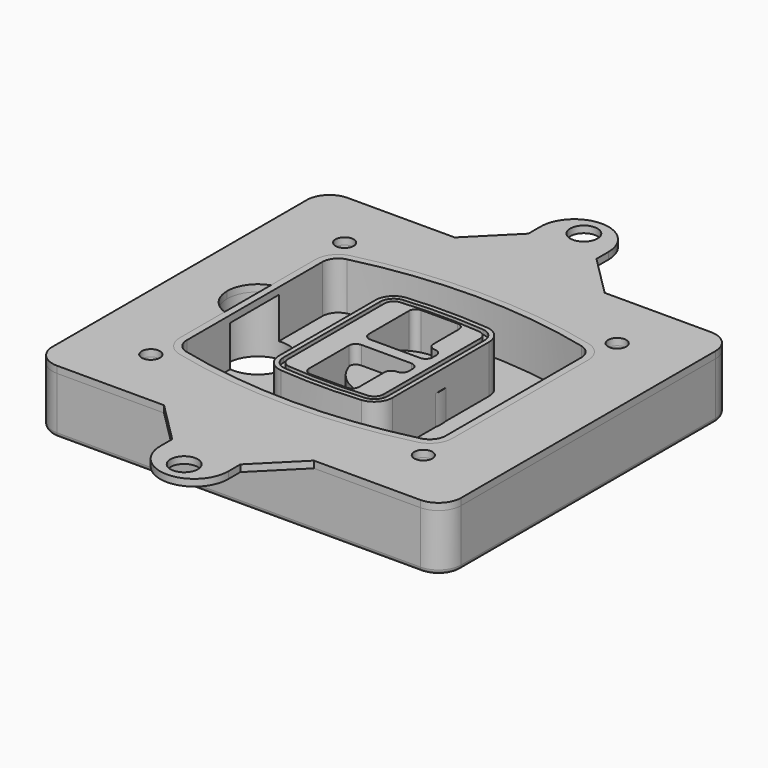
from build123d import *

# Parameters (mm, degrees)
F0_R      = 4
F1_DEPTH  = 25
F2_DEPTH  = 3
F3_DEPTH  = 18
F5_DEPTH  = 21
F6_DEPTH  = 2
F8_DEPTH  = 20
F9_DEPTH  = 16
F10_DEPTH = 25
F7_R      = 6
F7_R_2    = 4
F11_DEPTH = 6
F13_DEPTH = 9
F15_R     = 2
F16_R     = 6
F16_R_2   = 4
F17_DEPTH = 3


# Not quite as in the source:
# - a feature of the source that left no trace in its solid (it failed there, or was rolled back) is left out
# - a feature names something its author has since deleted; it is built from what else it names


with BuildPart() as f1:
    # F0 (on Top) → F1 (new body)
    with BuildSketch(Plane.XY):
        with BuildLine():
            ThreePointArc((-90, -70), (-87.0710678119, -77.0710678119), (-80, -80))
            Line((-80, -80), (80, -80))
            ThreePointArc((80, -80), (87.0710678119, -77.0710678119), (90, -70))
            Line((90, -70), (90, 70))
            ThreePointArc((90, 70), (87.0710678119, 77.0710678119), (80, 80))
            Line((80, 80), (-80, 80))
            ThreePointArc((-80, 80), (-87.0710678119, 77.0710678119), (-90, 70))
            Line((-90, 70), (-90, -70))
        make_face()
        with Locations((-60, -53.3333333333)):
            Circle(F0_R, mode=Mode.SUBTRACT)
        with Locations((60, -53.3333333333)):
            Circle(F0_R, mode=Mode.SUBTRACT)
        with Locations((-60, 53.3333333333)):
            Circle(F0_R, mode=Mode.SUBTRACT)
        with BuildLine():
            ThreePointArc((-64, 37.2990447398), (-61.0143011354, 45.9411029726), (-53.3306899286, 50.8970778549))
            ThreePointArc((-53.3306899286, 50.8970778549), (0, 57.3333333333), (53.3306899286, 50.8970778549))
            ThreePointArc((53.3306899286, 50.8970778549), (61.0143011354, 45.9411029726), (64, 37.2990447398))
            Line((64, 37.2990447398), (64, -37.2990447398))
            ThreePointArc((64, -37.2990447398), (61.0143011354, -45.9411029726), (53.3306899286, -50.8970778549))
            ThreePointArc((53.3306899286, -50.8970778549), (0, -57.3333333333), (-53.3306899286, -50.8970778549))
            ThreePointArc((-53.3306899286, -50.8970778549), (-61.0143011354, -45.9411029726), (-64, -37.2990447398))
            Line((-64, -37.2990447398), (-64, 37.2990447398))
        make_face(mode=Mode.SUBTRACT)
        with Locations((60, 53.3333333333)):
            Circle(F0_R, mode=Mode.SUBTRACT)
        with BuildLine():
            ThreePointArc((53.3306899286, 50.8970778549), (0, 57.3333333333), (-53.3306899286, 50.8970778549))
            ThreePointArc((-53.3306899286, 50.8970778549), (-61.0143011354, 45.9411029726), (-64, 37.2990447398))
            Line((-64, 37.2990447398), (-64, -37.2990447398))
            ThreePointArc((-64, -37.2990447398), (-61.0143011354, -45.9411029726), (-53.3306899286, -50.8970778549))
            ThreePointArc((-53.3306899286, -50.8970778549), (0, -57.3333333333), (53.3306899286, -50.8970778549))
            ThreePointArc((53.3306899286, -50.8970778549), (61.0143011354, -45.9411029726), (64, -37.2990447398))
            Line((64, -37.2990447398), (64, 37.2990447398))
            ThreePointArc((64, 37.2990447398), (61.0143011354, 45.9411029726), (53.3306899286, 50.8970778549))
        make_face()
        with BuildLine():
            Line((-60, -37.2990447398), (-60, 37.2990447398))
            ThreePointArc((-60, 37.2990447398), (-57.8673579538, 43.4719434775), (-52.3790642347, 47.0119255363))
            ThreePointArc((-52.3790642347, 47.0119255363), (0, 53.3333333333), (52.3790642347, 47.0119255363))
            ThreePointArc((52.3790642347, 47.0119255363), (57.8673579538, 43.4719434775), (60, 37.2990447398))
            Line((60, 37.2990447398), (60, -37.2990447398))
            ThreePointArc((60, -37.2990447398), (57.8673579538, -43.4719434775), (52.3790642347, -47.0119255363))
            ThreePointArc((52.3790642347, -47.0119255363), (0, -53.3333333333), (-52.3790642347, -47.0119255363))
            ThreePointArc((-52.3790642347, -47.0119255363), (-57.8673579538, -43.4719434775), (-60, -37.2990447398))
        make_face(mode=Mode.SUBTRACT)
        with BuildLine():
            ThreePointArc((-52.3790642347, 47.0119255363), (-57.8673579538, 43.4719434775), (-60, 37.2990447398))
            Line((-60, 37.2990447398), (-60, -37.2990447398))
            ThreePointArc((-60, -37.2990447398), (-57.8673579538, -43.4719434775), (-52.3790642347, -47.0119255363))
            ThreePointArc((-52.3790642347, -47.0119255363), (0, -53.3333333333), (52.3790642347, -47.0119255363))
            ThreePointArc((52.3790642347, -47.0119255363), (57.8673579538, -43.4719434775), (60, -37.2990447398))
            Line((60, -37.2990447398), (60, 37.2990447398))
            ThreePointArc((60, 37.2990447398), (57.8673579538, 43.4719434775), (52.3790642347, 47.0119255363))
            ThreePointArc((52.3790642347, 47.0119255363), (0, 53.3333333333), (-52.3790642347, 47.0119255363))
        make_face()
        with BuildLine():
            ThreePointArc((51.6653449643, 44.0980612973), (55.5071505677, 41.6200738562), (57, 37.2990447398))
            Line((57, 37.2990447398), (57, -37.2990447398))
            ThreePointArc((57, -37.2990447398), (55.5071505677, -41.6200738562), (51.6653449643, -44.0980612973))
            ThreePointArc((51.6653449643, -44.0980612973), (0, -50.3333333333), (-51.6653449643, -44.0980612973))
            ThreePointArc((-51.6653449643, -44.0980612973), (-55.5071505677, -41.6200738562), (-57, -37.2990447398))
            Line((-57, -37.2990447398), (-57, 37.2990447398))
            ThreePointArc((-57, 37.2990447398), (-55.5071505677, 41.6200738562), (-51.6653449643, 44.0980612973))
            ThreePointArc((-51.6653449643, 44.0980612973), (0, 50.3333333333), (51.6653449643, 44.0980612973))
        make_face(mode=Mode.SUBTRACT)
        with BuildLine():
            Line((57, -37.2990447398), (57, 37.2990447398))
            ThreePointArc((57, 37.2990447398), (55.5071505677, 41.6200738562), (51.6653449643, 44.0980612973))
            ThreePointArc((51.6653449643, 44.0980612973), (0, 50.3333333333), (-51.6653449643, 44.0980612973))
            ThreePointArc((-51.6653449643, 44.0980612973), (-55.5071505677, 41.6200738562), (-57, 37.2990447398))
            Line((-57, 37.2990447398), (-57, -37.2990447398))
            ThreePointArc((-57, -37.2990447398), (-55.5071505677, -41.6200738562), (-51.6653449643, -44.0980612973))
            ThreePointArc((-51.6653449643, -44.0980612973), (0, -50.3333333333), (51.6653449643, -44.0980612973))
            ThreePointArc((51.6653449643, -44.0980612973), (55.5071505677, -41.6200738562), (57, -37.2990447398))
        make_face()
    extrude(amount=-F1_DEPTH)

    # F0 (on Top) → F2 (join)
    with BuildSketch(Plane.XY):
        with BuildLine():
            ThreePointArc((-52.3790642347, 47.0119255363), (-57.8673579538, 43.4719434775), (-60, 37.2990447398))
            Line((-60, 37.2990447398), (-60, -37.2990447398))
            ThreePointArc((-60, -37.2990447398), (-57.8673579538, -43.4719434775), (-52.3790642347, -47.0119255363))
            ThreePointArc((-52.3790642347, -47.0119255363), (0, -53.3333333333), (52.3790642347, -47.0119255363))
            ThreePointArc((52.3790642347, -47.0119255363), (57.8673579538, -43.4719434775), (60, -37.2990447398))
            Line((60, -37.2990447398), (60, 37.2990447398))
            ThreePointArc((60, 37.2990447398), (57.8673579538, 43.4719434775), (52.3790642347, 47.0119255363))
            ThreePointArc((52.3790642347, 47.0119255363), (0, 53.3333333333), (-52.3790642347, 47.0119255363))
        make_face()
        with BuildLine():
            ThreePointArc((51.6653449643, 44.0980612973), (55.5071505677, 41.6200738562), (57, 37.2990447398))
            Line((57, 37.2990447398), (57, -37.2990447398))
            ThreePointArc((57, -37.2990447398), (55.5071505677, -41.6200738562), (51.6653449643, -44.0980612973))
            ThreePointArc((51.6653449643, -44.0980612973), (0, -50.3333333333), (-51.6653449643, -44.0980612973))
            ThreePointArc((-51.6653449643, -44.0980612973), (-55.5071505677, -41.6200738562), (-57, -37.2990447398))
            Line((-57, -37.2990447398), (-57, 37.2990447398))
            ThreePointArc((-57, 37.2990447398), (-55.5071505677, 41.6200738562), (-51.6653449643, 44.0980612973))
            ThreePointArc((-51.6653449643, 44.0980612973), (0, 50.3333333333), (51.6653449643, 44.0980612973))
        make_face(mode=Mode.SUBTRACT)
    extrude(amount=F2_DEPTH)

    # F0 (on Top) → F3 (cut)
    with BuildSketch(Plane.XY):
        with BuildLine():
            Line((57, -37.2990447398), (57, 37.2990447398))
            ThreePointArc((57, 37.2990447398), (55.5071505677, 41.6200738562), (51.6653449643, 44.0980612973))
            ThreePointArc((51.6653449643, 44.0980612973), (0, 50.3333333333), (-51.6653449643, 44.0980612973))
            ThreePointArc((-51.6653449643, 44.0980612973), (-55.5071505677, 41.6200738562), (-57, 37.2990447398))
            Line((-57, 37.2990447398), (-57, -37.2990447398))
            ThreePointArc((-57, -37.2990447398), (-55.5071505677, -41.6200738562), (-51.6653449643, -44.0980612973))
            ThreePointArc((-51.6653449643, -44.0980612973), (0, -50.3333333333), (51.6653449643, -44.0980612973))
            ThreePointArc((51.6653449643, -44.0980612973), (55.5071505677, -41.6200738562), (57, -37.2990447398))
        make_face()
    extrude(amount=-F3_DEPTH, mode=Mode.SUBTRACT)

    # F4 (on face) → F5 (join, through all)
    with BuildSketch(Plane.XY.offset(3)):
        with BuildLine():
            ThreePointArc((-25, -26.587695628), (-22.8992979869, -31.9912392117), (-17.7004291845, -34.5569740744))
            ThreePointArc((-17.7004291845, -34.5569740744), (0, -35.3333333333), (17.7004291845, -34.5569740744))
            ThreePointArc((17.7004291845, -34.5569740744), (22.8992979869, -31.9912392117), (25, -26.587695628))
            Line((25, -26.587695628), (25, 26.587695628))
            ThreePointArc((25, 26.587695628), (22.8992979869, 31.9912392117), (17.7004291845, 34.5569740744))
            ThreePointArc((17.7004291845, 34.5569740744), (0, 35.3333333333), (-17.7004291845, 34.5569740744))
            ThreePointArc((-17.7004291845, 34.5569740744), (-22.8992979869, 31.9912392117), (-25, 26.587695628))
            Line((-25, 26.587695628), (-25, -26.587695628))
        make_face()
        with BuildLine():
            ThreePointArc((17.5253218884, 32.5646544628), (21.4244734902, 30.6403533158), (23, 26.587695628))
            Line((23, 26.587695628), (23, -26.587695628))
            ThreePointArc((23, -26.587695628), (21.4244734902, -30.6403533158), (17.5253218884, -32.5646544628))
            ThreePointArc((17.5253218884, -32.5646544628), (0, -33.3333333333), (-17.5253218884, -32.5646544628))
            ThreePointArc((-17.5253218884, -32.5646544628), (-21.4244734902, -30.6403533158), (-23, -26.587695628))
            Line((-23, -26.587695628), (-23, 26.587695628))
            ThreePointArc((-23, 26.587695628), (-21.4244734902, 30.6403533158), (-17.5253218884, 32.5646544628))
            ThreePointArc((-17.5253218884, 32.5646544628), (0, 33.3333333333), (17.5253218884, 32.5646544628))
        make_face(mode=Mode.SUBTRACT)
        with BuildLine():
            Line((23, -26.587695628), (23, 26.587695628))
            ThreePointArc((23, 26.587695628), (21.4244734902, 30.6403533158), (17.5253218884, 32.5646544628))
            ThreePointArc((17.5253218884, 32.5646544628), (0, 33.3333333333), (-17.5253218884, 32.5646544628))
            ThreePointArc((-17.5253218884, 32.5646544628), (-21.4244734902, 30.6403533158), (-23, 26.587695628))
            Line((-23, 26.587695628), (-23, -26.587695628))
            ThreePointArc((-23, -26.587695628), (-21.4244734902, -30.6403533158), (-17.5253218884, -32.5646544628))
            ThreePointArc((-17.5253218884, -32.5646544628), (0, -33.3333333333), (17.5253218884, -32.5646544628))
            ThreePointArc((17.5253218884, -32.5646544628), (21.4244734902, -30.6403533158), (23, -26.587695628))
        make_face()
        with BuildLine():
            ThreePointArc((17.3502145923, 30.5723348512), (19.9496489934, 29.2894674198), (21, 26.587695628))
            Line((21, 26.587695628), (21, -26.587695628))
            ThreePointArc((21, -26.587695628), (19.9496489934, -29.2894674198), (17.3502145923, -30.5723348512))
            ThreePointArc((17.3502145923, -30.5723348512), (0, -31.3333333333), (-17.3502145923, -30.5723348512))
            ThreePointArc((-17.3502145923, -30.5723348512), (-19.9496489934, -29.2894674198), (-21, -26.587695628))
            Line((-21, -26.587695628), (-21, 26.587695628))
            ThreePointArc((-21, 26.587695628), (-19.9496489934, 29.2894674198), (-17.3502145923, 30.5723348512))
            ThreePointArc((-17.3502145923, 30.5723348512), (0, 31.3333333333), (17.3502145923, 30.5723348512))
        make_face(mode=Mode.SUBTRACT)
        with BuildLine():
            Line((21, -26.587695628), (21, 26.587695628))
            ThreePointArc((21, 26.587695628), (19.9496489934, 29.2894674198), (17.3502145923, 30.5723348512))
            ThreePointArc((17.3502145923, 30.5723348512), (0, 31.3333333333), (-17.3502145923, 30.5723348512))
            ThreePointArc((-17.3502145923, 30.5723348512), (-19.9496489934, 29.2894674198), (-21, 26.587695628))
            Line((-21, 26.587695628), (-21, -26.587695628))
            ThreePointArc((-21, -26.587695628), (-19.9496489934, -29.2894674198), (-17.3502145923, -30.5723348512))
            ThreePointArc((-17.3502145923, -30.5723348512), (0, -31.3333333333), (17.3502145923, -30.5723348512))
            ThreePointArc((17.3502145923, -30.5723348512), (19.9496489934, -29.2894674198), (21, -26.587695628))
        make_face()
        with BuildLine():
            Line((-8, -2.5), (14, -2.5))
            ThreePointArc((14, -2.5), (16.1213203436, -3.3786796564), (17, -5.5))
            Line((17, -5.5), (17, -7.5))
            ThreePointArc((17, -7.5), (16.1213203436, -9.6213203436), (14, -10.5))
            ThreePointArc((14, -10.5), (11.8786796564, -11.3786796564), (11, -13.5))
            Line((11, -13.5), (11, -27.5))
            ThreePointArc((11, -27.5), (10.1213203436, -29.6213203436), (8, -30.5))
            Line((8, -30.5), (-8, -30.5))
            ThreePointArc((-8, -30.5), (-10.1213203436, -29.6213203436), (-11, -27.5))
            Line((-11, -27.5), (-11, -5.5))
            ThreePointArc((-11, -5.5), (-10.1213203436, -3.3786796564), (-8, -2.5))
        make_face(mode=Mode.SUBTRACT)
        with BuildLine():
            ThreePointArc((-8, 2.5), (-10.1213203436, 3.3786796564), (-11, 5.5))
            Line((-11, 5.5), (-11, 27.5))
            ThreePointArc((-11, 27.5), (-10.1213203436, 29.6213203436), (-8, 30.5))
            Line((-8, 30.5), (8, 30.5))
            ThreePointArc((8, 30.5), (10.1213203436, 29.6213203436), (11, 27.5))
            Line((11, 27.5), (11, 13.5))
            ThreePointArc((11, 13.5), (11.8786796564, 11.3786796564), (14, 10.5))
            ThreePointArc((14, 10.5), (16.1213203436, 9.6213203436), (17, 7.5))
            Line((17, 7.5), (17, 5.5))
            ThreePointArc((17, 5.5), (16.1213203436, 3.3786796564), (14, 2.5))
            Line((14, 2.5), (-8, 2.5))
        make_face(mode=Mode.SUBTRACT)
    extrude(amount=-F5_DEPTH)

    # F4 (on face) → F6 (cut)
    with BuildSketch(Plane.XY.offset(3)):
        with BuildLine():
            Line((23, -26.587695628), (23, 26.587695628))
            ThreePointArc((23, 26.587695628), (21.4244734902, 30.6403533158), (17.5253218884, 32.5646544628))
            ThreePointArc((17.5253218884, 32.5646544628), (0, 33.3333333333), (-17.5253218884, 32.5646544628))
            ThreePointArc((-17.5253218884, 32.5646544628), (-21.4244734902, 30.6403533158), (-23, 26.587695628))
            Line((-23, 26.587695628), (-23, -26.587695628))
            ThreePointArc((-23, -26.587695628), (-21.4244734902, -30.6403533158), (-17.5253218884, -32.5646544628))
            ThreePointArc((-17.5253218884, -32.5646544628), (0, -33.3333333333), (17.5253218884, -32.5646544628))
            ThreePointArc((17.5253218884, -32.5646544628), (21.4244734902, -30.6403533158), (23, -26.587695628))
        make_face()
        with BuildLine():
            ThreePointArc((17.3502145923, 30.5723348512), (19.9496489934, 29.2894674198), (21, 26.587695628))
            Line((21, 26.587695628), (21, -26.587695628))
            ThreePointArc((21, -26.587695628), (19.9496489934, -29.2894674198), (17.3502145923, -30.5723348512))
            ThreePointArc((17.3502145923, -30.5723348512), (0, -31.3333333333), (-17.3502145923, -30.5723348512))
            ThreePointArc((-17.3502145923, -30.5723348512), (-19.9496489934, -29.2894674198), (-21, -26.587695628))
            Line((-21, -26.587695628), (-21, 26.587695628))
            ThreePointArc((-21, 26.587695628), (-19.9496489934, 29.2894674198), (-17.3502145923, 30.5723348512))
            ThreePointArc((-17.3502145923, 30.5723348512), (0, 31.3333333333), (17.3502145923, 30.5723348512))
        make_face(mode=Mode.SUBTRACT)
    extrude(amount=-F6_DEPTH, mode=Mode.SUBTRACT)

    # F7 (on face) → F8 (join)
    with BuildSketch(Plane(origin=(0, 0, -25), x_dir=(1, 0, 0), z_dir=(0, 0, -1))):
        with BuildLine():
            ThreePointArc((-6.71157564, 0), (6.7567035675, 13.4682792075), (20.224982775, 0))
            Line((20.224982775, 0), (25.224982775, 0))
            ThreePointArc((25.224982775, 0), (6.7567035675, 18.4682792075), (-11.71157564, 0))
            Line((-11.71157564, 0), (-6.71157564, 0))
        make_face()
        with BuildLine():
            Line((-6.71157564, 0), (20.224982775, 0))
            ThreePointArc((20.224982775, 0), (6.7567035675, 13.4682792075), (-6.71157564, 0))
        make_face()
        with BuildLine():
            ThreePointArc((-6.71157564, 0), (6.7567035675, -13.4682792075), (20.224982775, 0))
            Line((20.224982775, 0), (-6.71157564, 0))
        make_face()
        with BuildLine():
            Line((25.224982775, 0), (20.224982775, 0))
            ThreePointArc((20.224982775, 0), (6.7567035675, -13.4682792075), (-6.71157564, 0))
            Line((-6.71157564, 0), (-11.71157564, 0))
            ThreePointArc((-11.71157564, 0), (6.7567035675, -18.4682792075), (25.224982775, 0))
        make_face()
    extrude(amount=-F8_DEPTH)

    # F7 (on face) → F9 (cut)
    with BuildSketch(Plane(origin=(0, 0, -25), x_dir=(1, 0, 0), z_dir=(0, 0, -1))):
        with BuildLine():
            Line((-6.71157564, 0), (20.224982775, 0))
            ThreePointArc((20.224982775, 0), (6.7567035675, 13.4682792075), (-6.71157564, 0))
        make_face()
        with BuildLine():
            ThreePointArc((-6.71157564, 0), (6.7567035675, -13.4682792075), (20.224982775, 0))
            Line((20.224982775, 0), (-6.71157564, 0))
        make_face()
    extrude(amount=-F9_DEPTH, mode=Mode.SUBTRACT)

    # F7 (on face) → F10 (cut)
    with BuildSketch(Plane(origin=(0, 0, -25), x_dir=(1, 0, 0), z_dir=(0, 0, -1))):
        with BuildLine():
            Line((-69.0318229325, 0), (-42.0952645175, 0))
            ThreePointArc((-42.0952645175, 0), (-55.563543725, 13.4682792075), (-69.0318229325, 0))
        make_face()
        with BuildLine():
            ThreePointArc((-69.0318229325, 0), (-55.563543725, -13.4682792075), (-42.0952645175, 0))
            Line((-42.0952645175, 0), (-69.0318229325, 0))
        make_face()
    extrude(amount=-F10_DEPTH, mode=Mode.SUBTRACT)

    # F7 (on face) → F11 (cut)
    with BuildSketch(Plane(origin=(0, 0, -25), x_dir=(1, 0, 0), z_dir=(0, 0, -1))):
        with Locations((60, -53.3333333333)):
            Circle(F7_R)
        with Locations((60, -53.3333333333)):
            Circle(F7_R_2, mode=Mode.SUBTRACT)
        with Locations((-60, -53.3333333333)):
            Circle(F7_R)
        with Locations((-60, -53.3333333333)):
            Circle(F7_R_2, mode=Mode.SUBTRACT)
        with Locations((-60, 53.3333333333)):
            Circle(F7_R)
        with Locations((-60, 53.3333333333)):
            Circle(F7_R_2, mode=Mode.SUBTRACT)
        with Locations((60, 53.3333333333)):
            Circle(F7_R)
        with Locations((60, 53.3333333333)):
            Circle(F7_R_2, mode=Mode.SUBTRACT)
    extrude(amount=-F11_DEPTH, mode=Mode.SUBTRACT)

    # F12 (on face) → F13 (cut, through all)
    with BuildSketch(Plane(origin=(0, 0, -9), x_dir=(1, 0, 0), z_dir=(0, 0, -1))):
        with BuildLine():
            ThreePointArc((20.224982775, 0), (20.1663399806, 1.2554664788), (19.9909222755, 2.5))
            Line((19.9909222755, 2.5), (14, 2.5))
            ThreePointArc((14, 2.5), (16.1213203436, 3.3786796564), (17, 5.5))
            Line((17, 5.5), (17, 7.5))
            ThreePointArc((17, 7.5), (16.1213203436, 9.6213203436), (14, 10.5))
            ThreePointArc((14, 10.5), (12.1627255951, 11.1284134507), (11.0951631559, 12.750384826))
            ThreePointArc((11.0951631559, 12.750384826), (11.0476113807, 12.7664660322), (11, 12.7823698976))
            Line((11, 12.7823698976), (11, -12.7823698976))
            ThreePointArc((11, -12.7823698976), (11.0476113807, -12.7664660322), (11.0951631559, -12.750384826))
            ThreePointArc((11.0951631559, -12.750384826), (12.1627255951, -11.1284134507), (14, -10.5))
            ThreePointArc((14, -10.5), (16.1213203436, -9.6213203436), (17, -7.5))
            Line((17, -7.5), (17, -5.5))
            ThreePointArc((17, -5.5), (16.1213203436, -3.3786796564), (14, -2.5))
            Line((14, -2.5), (19.9909222755, -2.5))
            ThreePointArc((19.9909222755, -2.5), (20.1663399806, -1.2554664788), (20.224982775, 0))
        make_face()
    extrude(amount=F13_DEPTH, mode=Mode.SUBTRACT)

    # F15
    f15_edges = [f1.edges().sort_by_distance(p)[0] for p in [
        (0, -80, -25),
        (-87.071068, -77.071068, -25),
        (-90, 0, -25),
        (-87.071068, 77.071068, -25),
        (87.071068, -77.071068, -25),
        (0, 80, -25),
        (90, 0, -25),
        (87.071068, 77.071068, -25),
    ]]
    fillet(f15_edges, radius=F15_R)


with BuildPart() as f17:
    # F16 (on face) → F17 (new body, through all)
    with BuildSketch(Plane.XY):
        with BuildLine():
            Line((-14.8513905406, 98), (-32.8513905406, 80))
            Line((-32.8513905406, 80), (33.1457935262, 80))
            Line((33.1457935262, 80), (15.1457935262, 98))
            Line((15.1457935262, 98), (15.1457935262, 104.6209738977))
            ThreePointArc((15.1457935262, 104.6209738977), (0.0004680335, 119.6202698978), (-14.8513905406, 104.3303365535))
            Line((-14.8513905406, 104.3303365535), (-14.8513905406, 98))
        make_face()
        with Locations((0, 110)):
            Circle(F16_R, mode=Mode.SUBTRACT)
        with BuildLine():
            Line((33.1457935262, -80), (-32.8513905406, -80))
            Line((-32.8513905406, -80), (-14.8513905406, -98))
            Line((-14.8513905406, -98), (-14.8513905406, -104.3303365535))
            ThreePointArc((-14.8513905406, -104.3303365535), (0.0004680335, -119.6202698978), (15.1457935262, -104.6209738977))
            Line((15.1457935262, -104.6209738977), (15.1457935262, -98))
            Line((15.1457935262, -98), (33.1457935262, -80))
        make_face()
        with Locations((0, -110)):
            Circle(F16_R, mode=Mode.SUBTRACT)
        with BuildLine():
            Line((33.1457935262, 80), (-32.8513905406, 80))
            Line((-32.8513905406, 80), (-80, 80))
            ThreePointArc((-80, 80), (-87.0710678119, 77.0710678119), (-90, 70))
            Line((-90, 70), (-90, -70))
            ThreePointArc((-90, -70), (-87.0710678119, -77.0710678119), (-80, -80))
            Line((-80, -80), (-32.8513905406, -80))
            Line((-32.8513905406, -80), (33.1457935262, -80))
            Line((33.1457935262, -80), (80, -80))
            ThreePointArc((80, -80), (87.0710678119, -77.0710678119), (90, -70))
            Line((90, -70), (90, 70))
            ThreePointArc((90, 70), (87.0710678119, 77.0710678119), (80, 80))
            Line((80, 80), (33.1457935262, 80))
        make_face()
        with Locations((-60, -53.3333333333)):
            Circle(F16_R_2, mode=Mode.SUBTRACT)
        with BuildLine():
            Line((-60, 12.7166190685), (-60, 37.2990447398))
            ThreePointArc((-60, 37.2990447398), (-57.8673579538, 43.4719434775), (-52.3790642347, 47.0119255363))
            ThreePointArc((-52.3790642347, 47.0119255363), (0, 53.3333333333), (52.3790642347, 47.0119255363))
            ThreePointArc((52.3790642347, 47.0119255363), (57.8673579538, 43.4719434775), (60, 37.2990447398))
            Line((60, 37.2990447398), (60, -37.2990447398))
            ThreePointArc((60, -37.2990447398), (57.8673579538, -43.4719434775), (52.3790642347, -47.0119255363))
            ThreePointArc((52.3790642347, -47.0119255363), (0, -53.3333333333), (-52.3790642347, -47.0119255363))
            ThreePointArc((-52.3790642347, -47.0119255363), (-57.8673579538, -43.4719434775), (-60, -37.2990447398))
            Line((-60, -37.2990447398), (-60, -12.7166190685))
            ThreePointArc((-60, -12.7166190685), (-66.5441169481, -7.798817635), (-69.0318229325, 0))
            ThreePointArc((-69.0318229325, 0), (-66.5441169481, 7.798817635), (-60, 12.7166190685))
        make_face(mode=Mode.SUBTRACT)
        with Locations((60, -53.3333333333)):
            Circle(F16_R_2, mode=Mode.SUBTRACT)
        with Locations((-60, 53.3333333333)):
            Circle(F16_R_2, mode=Mode.SUBTRACT)
        with Locations((60, 53.3333333333)):
            Circle(F16_R_2, mode=Mode.SUBTRACT)
    extrude(amount=F17_DEPTH)


solid = Compound([f1.part, f17.part])
